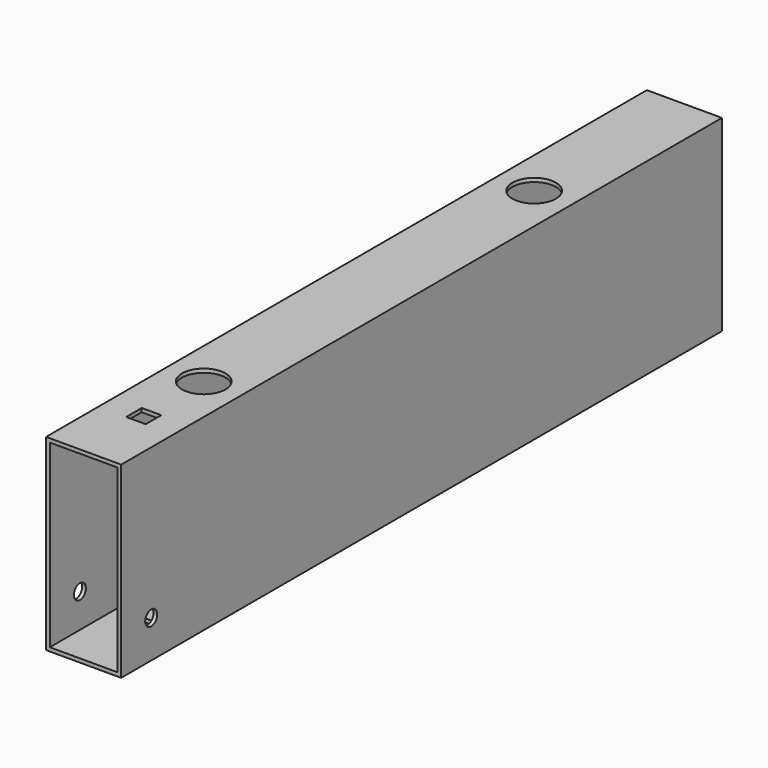
from build123d import *

# Parameters (mm, degrees)
F0_W     = 100
F0_H     = 250
F0_W_2   = 90
F0_H_2   = 240
F1_DEPTH = 1000
F2_R     = 10
F3_DEPTH = 100.001
F4_R     = 29
F5_R     = 29
F6_DEPTH = 5
F7_W     = 26
F7_H     = 26
F8_DEPTH = 250.001


# Not quite as in the source:
# - a feature names something its author has since deleted; it is built from what else it names


with BuildPart() as f1:
    # F0 (on Front) → F1 (new body)
    with BuildSketch(Plane.XZ):
        Rectangle(F0_W, F0_H)
        Rectangle(F0_W_2, F0_H_2, mode=Mode.SUBTRACT)
    extrude(amount=F1_DEPTH)

    # F2 (on face) → F3 (cut, through all)
    with BuildSketch(Plane.YZ.offset(50)):
        with Locations((-950, -75)):
            Circle(F2_R)
    extrude(amount=-F3_DEPTH, mode=Mode.SUBTRACT)

    # F4 (on face) + F5 (on face) → F6 (cut, through all)
    with BuildSketch(Plane.XY.offset(125)):
        with Locations((0, -800)):
            Circle(F4_R)
    with BuildSketch(Plane.XY.offset(125)):
        with Locations((0, -250)):
            Circle(F5_R)
    extrude(amount=-F6_DEPTH, mode=Mode.SUBTRACT)

    # F7 (on face) → F8 (cut, through all)
    with BuildSketch(Plane.XY.offset(125)):
        with Locations((0, -900)):
            Rectangle(F7_W, F7_H)
    extrude(amount=-F8_DEPTH, mode=Mode.SUBTRACT)


solid = f1.part
